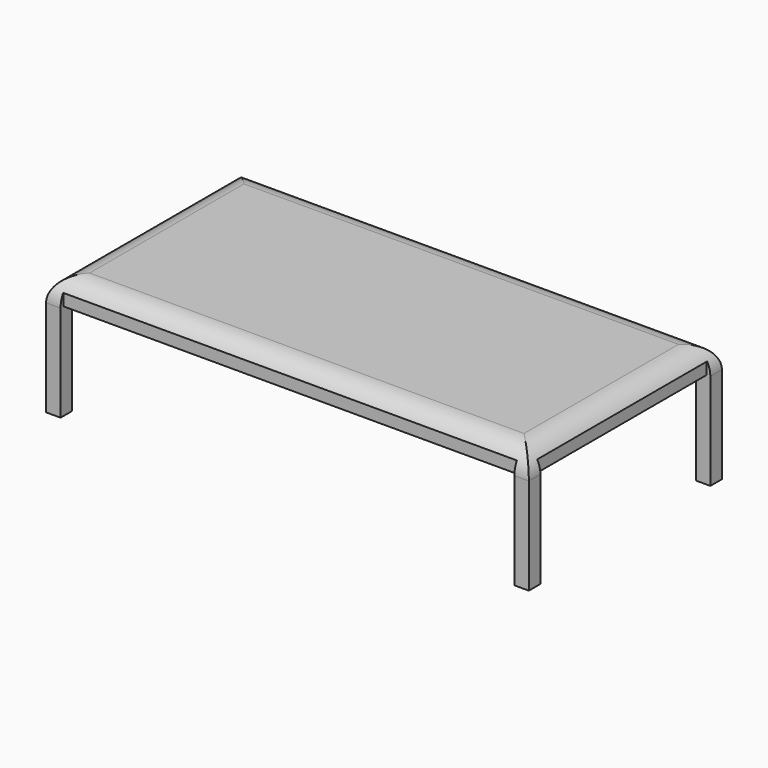
from build123d import *

# Parameters (mm, degrees)
F0_W         = 100
F0_H         = 50
F1_DEPTH     = 25
F3_W         = 44
F3_H         = 20
F4_DEPTH     = 100.001
F2_W         = 94
F2_H         = 20
F5_DEPTH     = 50.001
F6_W         = 94
F6_H         = 44
F6_H_2       = 0.75
F7_DEPTH     = 2.5
F8_DEPTH     = 3
F2_H_2       = 2.5
F9_DEPTH     = 0.75
F10_W        = 44
F10_H        = 2.5
F11_DEPTH    = 0.75
F13_DEPTH    = 0.75
F14_W        = 44
F14_H        = 2.5
F15_DEPTH    = 0.75
F16_W        = 44
F16_H        = 2.5
F17_DEPTH    = 0.75
F18_W        = 94
F18_H        = 2.5
F19_DEPTH    = 0.75
F20_W        = 94
F20_H        = 2.5
F21_DEPTH    = 0.75
F22_T1_DEPTH = 75
F22_T3_DEPTH = 125


# Not quite as in the source:
# - a fillet or chamfer that OpenCascade refuses, or shapes differently, is made with other operations: its cross-section is extruded or revolved along the edge and cut away or added


with BuildPart() as f1:
    # F0 (on Top) → F1 (new body)
    with BuildSketch(Plane.XY):
        with Locations((50, 25)):
            Rectangle(F0_W, F0_H)
    extrude(amount=F1_DEPTH)

    # F3 (on face) → F4 (cut, through all)
    with BuildSketch(Plane.YZ.offset(100)):
        with Locations((25, 10)):
            Rectangle(F3_W, F3_H)
    extrude(amount=-F4_DEPTH, mode=Mode.SUBTRACT)

    # F2 (on face) → F5 (cut, through all)
    with BuildSketch(Plane.XZ):
        with Locations((50, 10)):
            Rectangle(F2_W, F2_H)
    extrude(amount=-F5_DEPTH, mode=Mode.SUBTRACT)

    # F6 (on face) → F7 (cut)
    with BuildSketch(Plane(origin=(0, 0, 20), x_dir=(1, 0, 0), z_dir=(0, 0, -1))):
        with Locations((50, -25)):
            Rectangle(F6_W, F6_H)
        with Locations((50, -2.625)):
            Rectangle(F6_W, F6_H_2)
    extrude(amount=-F7_DEPTH, mode=Mode.SUBTRACT)

    # F6 (on face) → F8 (cut)
    with BuildSketch(Plane(origin=(0, 0, 20), x_dir=(1, 0, 0), z_dir=(0, 0, -1))):
        with Locations((50, -25)):
            Rectangle(F6_W, F6_H)
    extrude(amount=-F8_DEPTH, mode=Mode.SUBTRACT)

    # F2 (on face) → F9 (cut)
    with BuildSketch(Plane.XZ):
        with Locations((50, 21.25)):
            Rectangle(F2_W, F2_H_2)
    extrude(amount=-F9_DEPTH, mode=Mode.SUBTRACT)

    # F10 (on face) → F11 (cut)
    with BuildSketch(Plane(origin=(0, 0, 0), x_dir=(0, -1, 0), z_dir=(-1, 0, 0))):
        with Locations((-25, 21.25)):
            Rectangle(F10_W, F10_H)
    extrude(amount=-F11_DEPTH, mode=Mode.SUBTRACT)

    # F12 (on face) → F13 (cut)
    with BuildSketch(Plane.YZ.offset(3)):
        Polygon((3, 22.5), (3, 20), (47, 20), (47, 21.5), (47, 22.5), align=None)
    extrude(amount=-F13_DEPTH, mode=Mode.SUBTRACT)

    # F14 (on face) → F15 (cut)
    with BuildSketch(Plane.YZ.offset(100)):
        with Locations((25, 21.25)):
            Rectangle(F14_W, F14_H)
    extrude(amount=-F15_DEPTH, mode=Mode.SUBTRACT)

    # F16 (on face) → F17 (cut)
    with BuildSketch(Plane(origin=(97, 0, 0), x_dir=(0, -1, 0), z_dir=(-1, 0, 0))):
        with Locations((-25, 21.25)):
            Rectangle(F16_W, F16_H)
    extrude(amount=-F17_DEPTH, mode=Mode.SUBTRACT)

    # F18 (on face) → F19 (cut)
    with BuildSketch(Plane(origin=(0, 50, 0), x_dir=(-1, 0, 0), z_dir=(0, 1, 0))):
        with Locations((-50, 21.25)):
            Rectangle(F18_W, F18_H)
    extrude(amount=-F19_DEPTH, mode=Mode.SUBTRACT)

    # F20 (on face) → F21 (cut)
    with BuildSketch(Plane.XZ.offset(-47)):
        with Locations((50, 21.25)):
            Rectangle(F20_W, F20_H)
    extrude(amount=-F21_DEPTH, mode=Mode.SUBTRACT)

    # F22: fillet of radius 5 on 4 edges, made by hand

    # F22_s2 → F22_t1 (cut)
    with BuildSketch(Plane.XZ.offset(-62.5)):
        with BuildLine():
            ThreePointArc((0, 20), (1.4644660941, 23.5355339059), (5, 25))
            Line((5, 25), (0, 25))
            Line((0, 25), (0, 20))
        make_face()
        with BuildLine():
            ThreePointArc((100, 20), (98.5355339059, 23.5355339059), (95, 25))
            Line((95, 25), (100, 25))
            Line((100, 25), (100, 20))
        make_face()
    extrude(amount=F22_T1_DEPTH, mode=Mode.SUBTRACT)

    # F22_s4 → F22_t3 (cut)
    with BuildSketch(Plane.YZ.offset(-12.5)):
        with BuildLine():
            ThreePointArc((0, 20), (1.4644660941, 23.5355339059), (5, 25))
            Line((5, 25), (0, 25))
            Line((0, 25), (0, 20))
        make_face()
        with BuildLine():
            ThreePointArc((45, 25), (48.5355339059, 23.5355339059), (50, 20))
            Line((50, 20), (50, 25))
            Line((50, 25), (45, 25))
        make_face()
    extrude(amount=F22_T3_DEPTH, mode=Mode.SUBTRACT)


solid = f1.part
